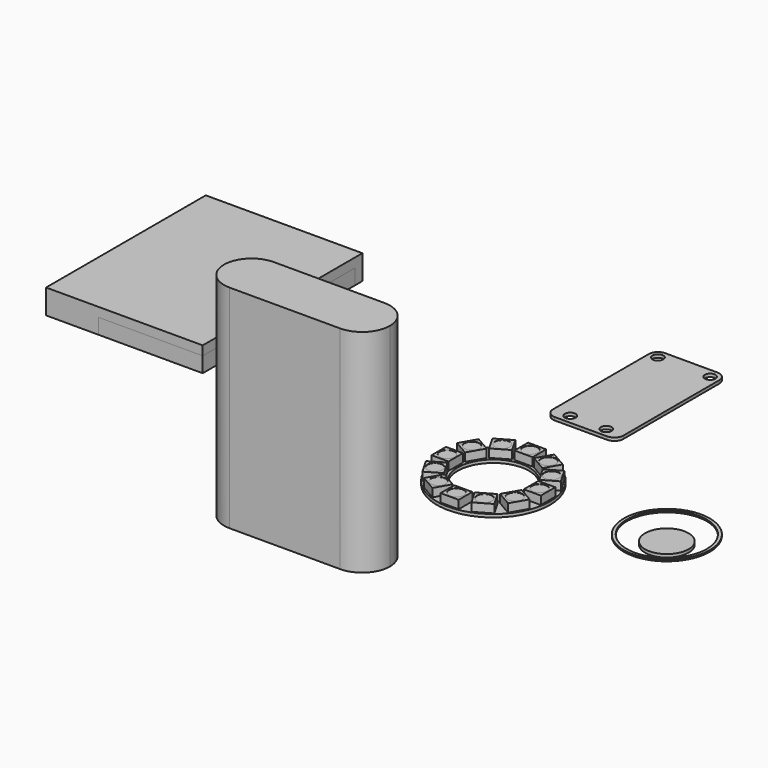
from build123d import *

# Parameters (mm, degrees)
F0_R      = 18.4
F0_W      = 5.8919586179
F0_H      = 5.543599081
F0_W_2    = 5.543599081
F0_H_2    = 5.8919586179
F0_R_2    = 11.65
F0_R_3    = 2.4221621224
F1_DEPTH  = 1
F2_DEPTH  = 2.7
F3_DEPTH  = 2.6
F4_R      = 0.75
F4_W      = 2.8461366892
F4_H      = 3.0996873975
F4_R_2    = 1.75
F4_R_3    = 0.6511885091
F5_DEPTH  = 1
F6_DEPTH  = 2
F7_R      = 7.085293516
F7_R_2    = 5.0696373744
F10_DEPTH = 1
F9_R      = 14
F9_R_2    = 13.0109775379
F11_DEPTH = 0.5
F13_R     = 1.75
F13_W     = 10.3073921055
F13_H     = 7.7943652868
F13_W_2   = 8.4696230255
F13_H_2   = 8.1840753555
F14_DEPTH = 1
F16_DEPTH = 69
F17_DEPTH = 69
F18_DEPTH = 69
F19_W     = 34
F19_H     = 60
F19_W_2   = 2
F20_DEPTH = 7
F19_H_2   = 2
F21_DEPTH = 8
F22_DEPTH = 5


# Not quite as in the source:
# - the program builds the solid bodies; features that only make, move or delete a surface that nothing else refers to are left out


with BuildPart() as f1:
    # F0 (on Top) → F1 (new body)
    with BuildSketch(Plane.XY):
        Circle(F0_R)
        with Locations((0, -15.025)):
            Rectangle(F0_W, F0_H, mode=Mode.SUBTRACT)
        Polygon((-6.3471068497, -16.8854701626), (-11.4496926908, -13.9394908537), (-8.6778931503, -9.1385932211), (-3.5753073092, -12.08457253), align=None, mode=Mode.SUBTRACT)
        Polygon((-13.9394908537, -11.4496926908), (-16.8854701626, -6.3471068497), (-12.08457253, -3.5753073092), (-9.1385932211, -8.6778931503), align=None, mode=Mode.SUBTRACT)
        Polygon((11.4496926908, -13.9394908537), (6.3471068497, -16.8854701626), (3.5753073092, -12.08457253), (8.6778931503, -9.1385932211), align=None, mode=Mode.SUBTRACT)
        Polygon((16.8854701626, -6.3471068497), (13.9394908537, -11.4496926908), (9.1385932211, -8.6778931503), (12.08457253, -3.5753073092), align=None, mode=Mode.SUBTRACT)
        with Locations((15.025, 0)):
            Rectangle(F0_W_2, F0_H_2, mode=Mode.SUBTRACT)
        with Locations((-15.025, 0)):
            Rectangle(F0_W_2, F0_H_2, mode=Mode.SUBTRACT)
        Polygon((-16.8854701626, 6.3471068497), (-13.9394908537, 11.4496926908), (-9.1385932211, 8.6778931503), (-12.08457253, 3.5753073092), align=None, mode=Mode.SUBTRACT)
        Polygon((-11.4496926908, 13.9394908537), (-6.3471068497, 16.8854701626), (-3.5753073092, 12.08457253), (-8.6778931503, 9.1385932211), align=None, mode=Mode.SUBTRACT)
        Circle(F0_R_2, mode=Mode.SUBTRACT)
        Polygon((13.9394908537, 11.4496926908), (16.8854701626, 6.3471068497), (12.08457253, 3.5753073092), (9.1385932211, 8.6778931503), align=None, mode=Mode.SUBTRACT)
        Polygon((6.3471068497, 16.8854701626), (11.4496926908, 13.9394908537), (8.6778931503, 9.1385932211), (3.5753073092, 12.08457253), align=None, mode=Mode.SUBTRACT)
        with Locations((0, 15.025)):
            Rectangle(F0_W, F0_H, mode=Mode.SUBTRACT)
        with Locations((0, -15.025)):
            Rectangle(F0_W, F0_H)
        with Locations((0, -15.025)):
            Circle(F0_R_3, mode=Mode.SUBTRACT)
        Polygon((3.5753073092, -12.08457253), (6.3471068497, -16.8854701626), (11.4496926908, -13.9394908537), (8.6778931503, -9.1385932211), align=None)
        with Locations((7.5125, -13.0120316919)):
            Circle(F0_R_3, mode=Mode.SUBTRACT)
        Polygon((9.1385932211, -8.6778931503), (13.9394908537, -11.4496926908), (16.8854701626, -6.3471068497), (12.08457253, -3.5753073092), align=None)
        with Locations((13.0120316919, -7.5125)):
            Circle(F0_R_3, mode=Mode.SUBTRACT)
        with Locations((15.025, 0)):
            Rectangle(F0_W_2, F0_H_2)
        with Locations((15.025, 0)):
            Circle(F0_R_3, mode=Mode.SUBTRACT)
        Polygon((-9.1385932211, 8.6778931503), (-13.9394908537, 11.4496926908), (-16.8854701626, 6.3471068497), (-12.08457253, 3.5753073092), align=None)
        with Locations((-13.0120316919, 7.5125)):
            Circle(F0_R_3, mode=Mode.SUBTRACT)
        with Locations((0, 15.025)):
            Rectangle(F0_W, F0_H)
        with Locations((0, 15.025)):
            Circle(F0_R_3, mode=Mode.SUBTRACT)
        with Locations((-15.025, 0)):
            Rectangle(F0_W_2, F0_H_2)
        with Locations((-15.025, 0)):
            Circle(F0_R_3, mode=Mode.SUBTRACT)
        Polygon((-3.5753073092, 12.08457253), (-6.3471068497, 16.8854701626), (-11.4496926908, 13.9394908537), (-8.6778931503, 9.1385932211), align=None)
        with Locations((-7.5125, 13.0120316919)):
            Circle(F0_R_3, mode=Mode.SUBTRACT)
        Polygon((12.08457253, 3.5753073092), (16.8854701626, 6.3471068497), (13.9394908537, 11.4496926908), (9.1385932211, 8.6778931503), align=None)
        with Locations((13.0120316919, 7.5125)):
            Circle(F0_R_3, mode=Mode.SUBTRACT)
        Polygon((-12.08457253, -3.5753073092), (-16.8854701626, -6.3471068497), (-13.9394908537, -11.4496926908), (-9.1385932211, -8.6778931503), align=None)
        with Locations((-13.0120316919, -7.5125)):
            Circle(F0_R_3, mode=Mode.SUBTRACT)
        Polygon((8.6778931503, 9.1385932211), (11.4496926908, 13.9394908537), (6.3471068497, 16.8854701626), (3.5753073092, 12.08457253), align=None)
        with Locations((7.5125, 13.0120316919)):
            Circle(F0_R_3, mode=Mode.SUBTRACT)
        Polygon((-8.6778931503, -9.1385932211), (-11.4496926908, -13.9394908537), (-6.3471068497, -16.8854701626), (-3.5753073092, -12.08457253), align=None)
        with Locations((-7.5125, -13.0120316919)):
            Circle(F0_R_3, mode=Mode.SUBTRACT)
        with Locations((0, 15.025)):
            Circle(F0_R_3)
        with Locations((-7.5125, 13.0120316919)):
            Circle(F0_R_3)
        with Locations((-13.0120316919, 7.5125)):
            Circle(F0_R_3)
        with Locations((-15.025, 0)):
            Circle(F0_R_3)
        with Locations((-13.0120316919, -7.5125)):
            Circle(F0_R_3)
        with Locations((-7.5125, -13.0120316919)):
            Circle(F0_R_3)
        with Locations((0, -15.025)):
            Circle(F0_R_3)
        with Locations((7.5125, -13.0120316919)):
            Circle(F0_R_3)
        with Locations((13.0120316919, -7.5125)):
            Circle(F0_R_3)
        with Locations((15.025, 0)):
            Circle(F0_R_3)
        with Locations((13.0120316919, 7.5125)):
            Circle(F0_R_3)
        with Locations((7.5125, 13.0120316919)):
            Circle(F0_R_3)
    extrude(amount=-F1_DEPTH)

    # F0 (on Top) → F2 (join)
    with BuildSketch(Plane.XY):
        Polygon((-9.1385932211, 8.6778931503), (-13.9394908537, 11.4496926908), (-16.8854701626, 6.3471068497), (-12.08457253, 3.5753073092), align=None)
        with Locations((-13.0120316919, 7.5125)):
            Circle(F0_R_3, mode=Mode.SUBTRACT)
        Polygon((-3.5753073092, 12.08457253), (-6.3471068497, 16.8854701626), (-11.4496926908, 13.9394908537), (-8.6778931503, 9.1385932211), align=None)
        with Locations((-7.5125, 13.0120316919)):
            Circle(F0_R_3, mode=Mode.SUBTRACT)
        with Locations((0, 15.025)):
            Rectangle(F0_W, F0_H)
        with Locations((0, 15.025)):
            Circle(F0_R_3, mode=Mode.SUBTRACT)
        Polygon((8.6778931503, 9.1385932211), (11.4496926908, 13.9394908537), (6.3471068497, 16.8854701626), (3.5753073092, 12.08457253), align=None)
        with Locations((7.5125, 13.0120316919)):
            Circle(F0_R_3, mode=Mode.SUBTRACT)
        Polygon((12.08457253, 3.5753073092), (16.8854701626, 6.3471068497), (13.9394908537, 11.4496926908), (9.1385932211, 8.6778931503), align=None)
        with Locations((13.0120316919, 7.5125)):
            Circle(F0_R_3, mode=Mode.SUBTRACT)
        with Locations((15.025, 0)):
            Rectangle(F0_W_2, F0_H_2)
        with Locations((15.025, 0)):
            Circle(F0_R_3, mode=Mode.SUBTRACT)
        with Locations((-15.025, 0)):
            Rectangle(F0_W_2, F0_H_2)
        with Locations((-15.025, 0)):
            Circle(F0_R_3, mode=Mode.SUBTRACT)
        Polygon((-12.08457253, -3.5753073092), (-16.8854701626, -6.3471068497), (-13.9394908537, -11.4496926908), (-9.1385932211, -8.6778931503), align=None)
        with Locations((-13.0120316919, -7.5125)):
            Circle(F0_R_3, mode=Mode.SUBTRACT)
        Polygon((9.1385932211, -8.6778931503), (13.9394908537, -11.4496926908), (16.8854701626, -6.3471068497), (12.08457253, -3.5753073092), align=None)
        with Locations((13.0120316919, -7.5125)):
            Circle(F0_R_3, mode=Mode.SUBTRACT)
        Polygon((3.5753073092, -12.08457253), (6.3471068497, -16.8854701626), (11.4496926908, -13.9394908537), (8.6778931503, -9.1385932211), align=None)
        with Locations((7.5125, -13.0120316919)):
            Circle(F0_R_3, mode=Mode.SUBTRACT)
        with Locations((0, -15.025)):
            Rectangle(F0_W, F0_H)
        with Locations((0, -15.025)):
            Circle(F0_R_3, mode=Mode.SUBTRACT)
        Polygon((-8.6778931503, -9.1385932211), (-11.4496926908, -13.9394908537), (-6.3471068497, -16.8854701626), (-3.5753073092, -12.08457253), align=None)
        with Locations((-7.5125, -13.0120316919)):
            Circle(F0_R_3, mode=Mode.SUBTRACT)
    extrude(amount=F2_DEPTH)

    # F0 (on Top) → F3 (join)
    with BuildSketch(Plane.XY):
        with Locations((-13.0120316919, 7.5125)):
            Circle(F0_R_3)
        with Locations((-7.5125, 13.0120316919)):
            Circle(F0_R_3)
        with Locations((0, 15.025)):
            Circle(F0_R_3)
        with Locations((7.5125, 13.0120316919)):
            Circle(F0_R_3)
        with Locations((13.0120316919, 7.5125)):
            Circle(F0_R_3)
        with Locations((15.025, 0)):
            Circle(F0_R_3)
        with Locations((13.0120316919, -7.5125)):
            Circle(F0_R_3)
        with Locations((0, -15.025)):
            Circle(F0_R_3)
        with Locations((-7.5125, -13.0120316919)):
            Circle(F0_R_3)
        with Locations((-13.0120316919, -7.5125)):
            Circle(F0_R_3)
        with Locations((-15.025, 0)):
            Circle(F0_R_3)
        with Locations((7.5125, -13.0120316919)):
            Circle(F0_R_3)
    extrude(amount=F3_DEPTH)


with BuildPart() as f5:
    # F4 (on Top) → F5 (new body)
    with BuildSketch(Plane.XY):
        with BuildLine():
            ThreePointArc((-84.2555893898, 3), (-83.3769097334, 0.8786796564), (-81.2555893898, 0))
            Line((-81.2555893898, 0), (-69.4555893898, 0))
            ThreePointArc((-69.4555893898, 0), (-67.3342690462, 0.8786796564), (-66.4555893898, 3))
            Line((-66.4555893898, 3), (-66.4555893898, 16.4))
            ThreePointArc((-66.4555893898, 16.4), (-67.3342690462, 18.5213203436), (-69.4555893898, 19.4))
            Line((-69.4555893898, 19.4), (-81.2555893898, 19.4))
            ThreePointArc((-81.2555893898, 19.4), (-83.3769097334, 18.5213203436), (-84.2555893898, 16.4))
            Line((-84.2555893898, 16.4), (-84.2555893898, 3))
        make_face()
        with Locations((-81.9555893898, 2.3430765141)):
            Circle(F4_R, mode=Mode.SUBTRACT)
        with Locations((-79.7555893898, 2.3430765141)):
            Circle(F4_R, mode=Mode.SUBTRACT)
        with Locations((-77.5555893898, 2.3430765141)):
            Circle(F4_R, mode=Mode.SUBTRACT)
        with Locations((-75.3555893898, 2.3430765141)):
            Circle(F4_R, mode=Mode.SUBTRACT)
        with Locations((-73.1555893898, 2.3430765141)):
            Circle(F4_R, mode=Mode.SUBTRACT)
        with Locations((-70.9555893898, 2.3430765141)):
            Circle(F4_R, mode=Mode.SUBTRACT)
        with Locations((-68.7555893898, 2.3430765141)):
            Circle(F4_R, mode=Mode.SUBTRACT)
        with Locations((-75.3555893898, 8.0819614232)):
            Rectangle(F4_W, F4_H, mode=Mode.SUBTRACT)
        with Locations((-80.7391181588, 15.8931782246)):
            Circle(F4_R_2, mode=Mode.SUBTRACT)
        with Locations((-77.0134851336, 14.8214334622)):
            Circle(F4_R_3, mode=Mode.SUBTRACT)
        with Locations((-73.697693646, 14.8214334622)):
            Circle(F4_R_3, mode=Mode.SUBTRACT)
        with Locations((-69.9720606208, 15.8931782246)):
            Circle(F4_R_2, mode=Mode.SUBTRACT)
    extrude(amount=F5_DEPTH)

    # F4 (on Top) → F6 (join)
    with BuildSketch(Plane.XY):
        with Locations((-75.3555893898, 8.0819614232)):
            Rectangle(F4_W, F4_H)
    extrude(amount=F6_DEPTH)


with BuildPart() as f10:
    # F7 (on Top) → F10 (new body)
    with BuildSketch(Plane.XY):
        with Locations((56.480774566, 0)):
            Circle(F7_R)
        with Locations((56.480774566, 0)):
            Circle(F7_R_2, mode=Mode.SUBTRACT)
        with Locations((56.480774566, 0)):
            Circle(F7_R_2)
    extrude(amount=F10_DEPTH)


with BuildPart() as f11:
    # F9 (on offset) → F11 (new body)
    with BuildSketch(Plane.XY.offset(2.5)):
        with Locations((56.480774566, 0)):
            Circle(F9_R)
        with Locations((56.480774566, 0)):
            Circle(F9_R_2, mode=Mode.SUBTRACT)
    extrude(amount=F11_DEPTH)


with BuildPart() as f14:
    # F13 (on Top) → F14 (new body)
    with BuildSketch(Plane.XY):
        with BuildLine():
            ThreePointArc((-11.5, 38.6043675244), (-10.6213203436, 36.4830471808), (-8.5, 35.6043675244))
            Line((-8.5, 35.6043675244), (8.5, 35.6043675244))
            ThreePointArc((8.5, 35.6043675244), (10.6213203436, 36.4830471808), (11.5, 38.6043675244))
            Line((11.5, 38.6043675244), (11.5, 62.1646121144))
            Line((11.5, 62.1646121144), (3.0303769745, 62.1646121144))
            Line((3.0303769745, 62.1646121144), (3.0303769745, 70.34868747))
            Line((3.0303769745, 70.34868747), (11.5, 70.34868747))
            Line((11.5, 70.34868747), (11.5, 77.6043675244))
            ThreePointArc((11.5, 77.6043675244), (10.6213203436, 79.7256878679), (8.5, 80.6043675244))
            Line((8.5, 80.6043675244), (-8.5, 80.6043675244))
            ThreePointArc((-8.5, 80.6043675244), (-10.6213203436, 79.7256878679), (-11.5, 77.6043675244))
            Line((-11.5, 77.6043675244), (-11.5, 38.6043675244))
        make_face()
        with Locations((-5.8610606939, 38.6043675244)):
            Circle(F13_R, mode=Mode.SUBTRACT)
        with Locations((5.8610606939, 38.6043675244)):
            Circle(F13_R, mode=Mode.SUBTRACT)
        with Locations((-8.5, 77.6043675244)):
            Circle(F13_R, mode=Mode.SUBTRACT)
        with Locations((0, 76.681599021)):
            Rectangle(F13_W, F13_H, mode=Mode.SUBTRACT)
        with Locations((8.5, 77.6043675244)):
            Circle(F13_R, mode=Mode.SUBTRACT)
        with Locations((0, 76.681599021)):
            Rectangle(F13_W, F13_H)
        with Locations((7.2651884872, 66.2566497922)):
            Rectangle(F13_W_2, F13_H_2)
    extrude(amount=F14_DEPTH)


with BuildPart() as f16:
    # F15 (on Top) → F16 (new body)
    with BuildSketch(Plane.XY):
        with BuildLine():
            ThreePointArc((0, -62.3885793499), (6.3639610307, -59.7525403806), (9, -53.3885793499))
            ThreePointArc((9, -53.3885793499), (6.3639610307, -47.0246183193), (0, -44.3885793499))
            ThreePointArc((0, -44.3885793499), (-9, -53.3885793499), (0, -62.3885793499))
        make_face()
    extrude(amount=F16_DEPTH)


with BuildPart() as f17:
    # F15 (on Top) → F17 (new body)
    with BuildSketch(Plane.XY):
        with BuildLine():
            ThreePointArc((-10, -53.3885793499), (-12.6137545303, -47.0469810655), (-18.9368597335, -44.3888008356))
            Line((-18.9368597335, -44.3888008356), (-19.06335079, -44.3888023151))
            ThreePointArc((-19.06335079, -44.3888023151), (-24.2400754876, -46.0713661588), (-27.5, -50.4305394584))
            ThreePointArc((-27.5, -50.4305394584), (-27.1258803254, -51.8885793499), (-27, -53.3885793499))
            ThreePointArc((-27, -53.3885793499), (-27.1258803254, -54.8885793499), (-27.5, -56.3466192415))
            ThreePointArc((-27.5, -56.3466192415), (-24.2142900105, -60.7241897326), (-18.999999959, -62.3885793499))
            ThreePointArc((-18.999999959, -62.3885793499), (-12.6360389548, -59.7525403661), (-10, -53.3885793499))
        make_face()
        with BuildLine():
            ThreePointArc((0, -62.3885793499), (-9, -53.3885793499), (0, -44.3885793499))
            Line((0, -44.3885793493), (-18.9368597335, -44.3888008356))
            ThreePointArc((-18.9368597335, -44.3888008356), (-12.6137545303, -47.0469810655), (-10, -53.3885793499))
            ThreePointArc((-10, -53.3885793499), (-12.6360389548, -59.7525403661), (-18.999999959, -62.3885793499))
            Line((-18.999999959, -62.3885793499), (0, -62.3885793499))
        make_face()
        with BuildLine():
            ThreePointArc((-27.5, -50.4305394584), (-28, -53.3885793499), (-27.5, -56.3466192415))
            ThreePointArc((-27.5, -56.3466192415), (-27.1258803254, -54.8885793499), (-27, -53.3885793499))
            ThreePointArc((-27, -53.3885793499), (-27.1258803254, -51.8885793499), (-27.5, -50.4305394584))
        make_face()
        with BuildLine():
            ThreePointArc((0, -62.3885793499), (6.3639610307, -59.7525403806), (9, -53.3885793499))
            ThreePointArc((9, -53.3885793499), (6.3639610307, -47.0246183193), (0, -44.3885793499))
            ThreePointArc((0, -44.3885793499), (-9, -53.3885793499), (0, -62.3885793499))
        make_face()
    extrude(amount=F17_DEPTH)


with BuildPart() as f18:
    # F15 (on Top) → F18 (new body)
    with BuildSketch(Plane.XY):
        with BuildLine():
            ThreePointArc((0, -62.3885793499), (6.3639610307, -59.7525403806), (9, -53.3885793499))
            ThreePointArc((9, -53.3885793499), (6.3639610307, -47.0246183193), (0, -44.3885793499))
            ThreePointArc((0, -44.3885793499), (-9, -53.3885793499), (0, -62.3885793499))
        make_face()
        with BuildLine():
            ThreePointArc((0, -62.3885793499), (-9, -53.3885793499), (0, -44.3885793499))
            Line((0, -44.3885793493), (-18.9368597335, -44.3888008356))
            ThreePointArc((-18.9368597335, -44.3888008356), (-12.6137545303, -47.0469810655), (-10, -53.3885793499))
            ThreePointArc((-10, -53.3885793499), (-12.6360389548, -59.7525403661), (-18.999999959, -62.3885793499))
            Line((-18.999999959, -62.3885793499), (0, -62.3885793499))
        make_face()
        with BuildLine():
            ThreePointArc((-10, -53.3885793499), (-12.6137545303, -47.0469810655), (-18.9368597335, -44.3888008356))
            Line((-18.9368597335, -44.3888008356), (-19.06335079, -44.3888023151))
            ThreePointArc((-19.06335079, -44.3888023151), (-24.2400754876, -46.0713661588), (-27.5, -50.4305394584))
            ThreePointArc((-27.5, -50.4305394584), (-27.1258803254, -51.8885793499), (-27, -53.3885793499))
            ThreePointArc((-27, -53.3885793499), (-27.1258803254, -54.8885793499), (-27.5, -56.3466192415))
            ThreePointArc((-27.5, -56.3466192415), (-24.2142900105, -60.7241897326), (-18.999999959, -62.3885793499))
            ThreePointArc((-18.999999959, -62.3885793499), (-12.6360389548, -59.7525403661), (-10, -53.3885793499))
        make_face()
        with BuildLine():
            ThreePointArc((-27.5, -50.4305394584), (-24.2400754876, -46.0713661588), (-19.06335079, -44.3888023151))
            Line((-19.06335079, -44.3888023151), (-35.9130486246, -44.3889993898))
            ThreePointArc((-35.9130486246, -44.3889993898), (-30.7503347649, -46.0782431799), (-27.5, -50.4305394584))
        make_face()
        with BuildLine():
            ThreePointArc((-36.000000041, -62.3885793499), (-30.7857099895, -60.7241897326), (-27.5, -56.3466192415))
            ThreePointArc((-27.5, -56.3466192415), (-28, -53.3885793499), (-27.5, -50.4305394584))
            ThreePointArc((-27.5, -50.4305394584), (-30.7503347649, -46.0782431799), (-35.9130486246, -44.3889993898))
            ThreePointArc((-35.9130486246, -44.3889993898), (-44.9998949893, -53.3451031345), (-36.000000041, -62.3885793499))
        make_face()
        with BuildLine():
            Line((-36.000000041, -62.3885793499), (-18.999999959, -62.3885793499))
            ThreePointArc((-18.999999959, -62.3885793499), (-24.2142900105, -60.7241897326), (-27.5, -56.3466192415))
            ThreePointArc((-27.5, -56.3466192415), (-30.7857099895, -60.7241897326), (-36.000000041, -62.3885793499))
        make_face()
        with BuildLine():
            ThreePointArc((-27.5, -50.4305394584), (-28, -53.3885793499), (-27.5, -56.3466192415))
            ThreePointArc((-27.5, -56.3466192415), (-27.1258803254, -54.8885793499), (-27, -53.3885793499))
            ThreePointArc((-27, -53.3885793499), (-27.1258803254, -51.8885793499), (-27.5, -50.4305394584))
        make_face()
    extrude(amount=F18_DEPTH)


with BuildPart() as f20:
    # F19 (on Top) → F20 (new body)
    with BuildSketch(Plane.XY):
        with Locations((-111.657017827, 30)):
            Rectangle(F19_W, F19_H)
        with Locations((-129.657017827, 30)):
            Rectangle(F19_W_2, F19_H)
    extrude(amount=F20_DEPTH)


with BuildPart() as f21:
    # F19 (on Top) → F21 (new body)
    with BuildSketch(Plane.XY):
        Polygon((-145.657017827, 0), (-130.657017827, 0), (-130.657017827, 60), (-128.657017827, 60), (-128.657017827, 62), (-94.657017827, 62), (-94.657017827, 65), (-145.657017827, 65), align=None)
        with Locations((-111.657017827, 61)):
            Rectangle(F19_W, F19_H_2)
        with Locations((-111.657017827, 30)):
            Rectangle(F19_W, F19_H)
        with Locations((-129.657017827, 30)):
            Rectangle(F19_W_2, F19_H)
    extrude(amount=F21_DEPTH)


with BuildPart() as f22:
    # F19 (on Top) → F22 (new body)
    with BuildSketch(Plane.XY):
        with Locations((-111.657017827, 30)):
            Rectangle(F19_W, F19_H)
        with Locations((-111.657017827, 61)):
            Rectangle(F19_W, F19_H_2)
    extrude(amount=F22_DEPTH)


solid = Compound([f1.part, f5.part, f10.part, f11.part, f14.part, f16.part, f17.part, f18.part, f20.part, f21.part, f22.part])
